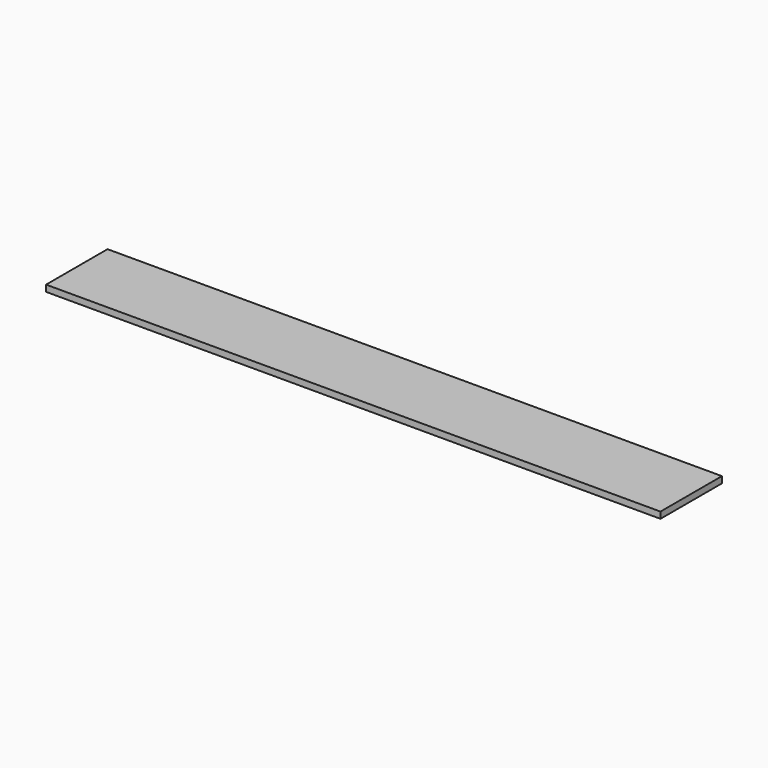
from build123d import *

# Parameters (mm, degrees)
F1_W     = 609.6
F1_H     = 76.2
F2_DEPTH = 6.35


# Not quite as in the source:
# - a variable given as a bare number and used for a length is read in inches; the dataset says mm whatever the document's units were


with BuildPart() as f2:
    # F1 (on Top) → F2 (new body)
    with BuildSketch(Plane.XY):
        with Locations((304.8, 38.1)):
            Rectangle(F1_W, F1_H)
    extrude(amount=F2_DEPTH)


solid = f2.part
